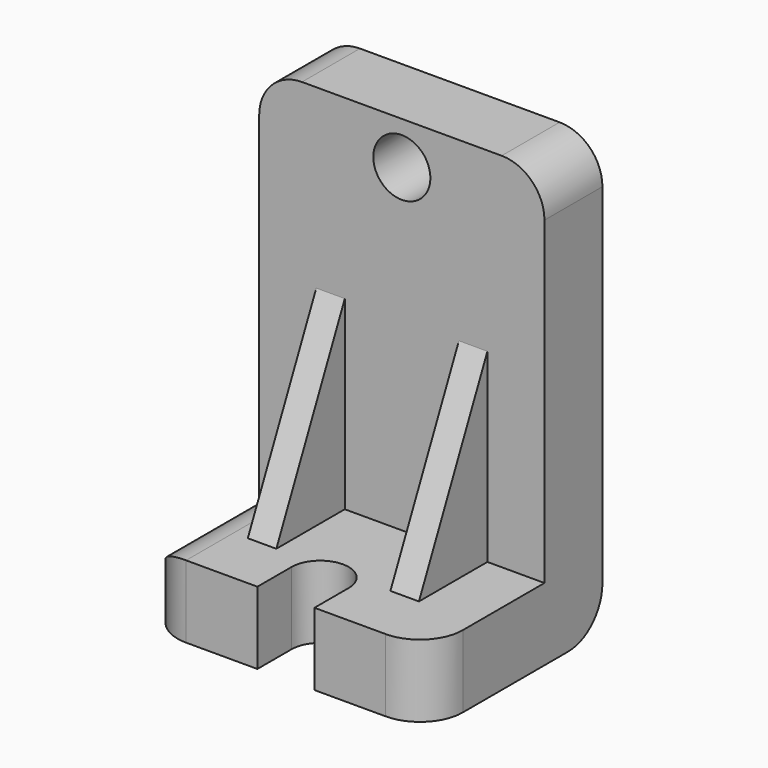
from build123d import *

# Parameters (mm, degrees)
F1_DEPTH = 50
F4_DEPTH = 25.401
F2_R     = 10
F5_DEPTH = 76.201
F8_DEPTH = 5
F11_R    = 15


# Not quite as in the source:
# - a feature of the source that left no trace in its solid (it failed there, or was rolled back) is left out
# - a pattern or mirror of a feature is missing from the dataset's text; its kind, count and spacing are read off the source's solid


with BuildPart() as f1:
    # F0 (on Right) → F1 (new body, symmetric)
    with BuildSketch(Plane.YZ):
        Polygon((-76.2, 0), (0, 0), (0, 152.4), (-25.4, 152.4), (-25.4, 25.4), (-76.2, 25.4), align=None)
    extrude(amount=F1_DEPTH, both=True)

    # F3 (on face) → F4 (cut, through all)
    with BuildSketch(Plane.XY.offset(25.4)):
        with BuildLine():
            ThreePointArc((-10, -61.2), (0, -71.2), (10, -61.2))
            ThreePointArc((10, -61.2), (0, -51.2), (-10, -61.2))
        make_face()
        with BuildLine():
            Line((10, -76.2), (10, -61.2))
            ThreePointArc((10, -61.2), (0, -71.2), (-10, -61.2))
            Line((-10, -61.2), (-10, -76.2))
            Line((-10, -76.2), (10, -76.2))
        make_face()
    extrude(amount=-F4_DEPTH, mode=Mode.SUBTRACT)

    # F2 (on face) → F5 (cut, through all)
    with BuildSketch(Plane(origin=(0, 0, 0), x_dir=(-1, 0, 0), z_dir=(0, 1, 0))):
        with Locations((0, 137.4)):
            Circle(F2_R)
    extrude(amount=-F5_DEPTH, mode=Mode.SUBTRACT)

    # F7 (on offset) → F8 (join, symmetric)
    with BuildSketch(Plane.YZ.offset(25)):
        Polygon((-25.4, 25.4), (-25.4, 90.4), (-55.4, 25.4), align=None)
    f8 = extrude(amount=F8_DEPTH, both=True)

    # F8_copies: F8 across plane
    add(f8.mirror(Plane(origin=(0, 0, 0), x_dir=(0, 0, -1), z_dir=(-1, 0, 0))))

    # F11 (call 1 of 5: OpenCascade refuses the feature's edges together)
    f11_edges = [f1.edges().sort_by_distance(p)[0] for p in [
        (-50, -12.7, 152.4),
    ]]
    fillet(f11_edges, radius=F11_R)

    # F11#2 (call 2 of 5)
    f11_2_edges = [f1.edges().sort_by_distance(p)[0] for p in [
        (50, -12.7, 152.4),
    ]]
    fillet(f11_2_edges, radius=F11_R)

    # F11#3 (call 3 of 5)
    f11_3_edges = [f1.edges().sort_by_distance(p)[0] for p in [
        (0, 0, 0),
    ]]
    fillet(f11_3_edges, radius=F11_R)

    # F11#4 (call 4 of 5)
    f11_4_edges = [f1.edges().sort_by_distance(p)[0] for p in [
        (50, -76.2, 12.7),
    ]]
    fillet(f11_4_edges, radius=F11_R)

    # F11#5 (call 5 of 5)
    f11_5_edges = [f1.edges().sort_by_distance(p)[0] for p in [
        (-50, -76.2, 12.7),
        (-50, -50.8, 25.4),
    ]]
    fillet(f11_5_edges, radius=F11_R)


solid = f1.part
